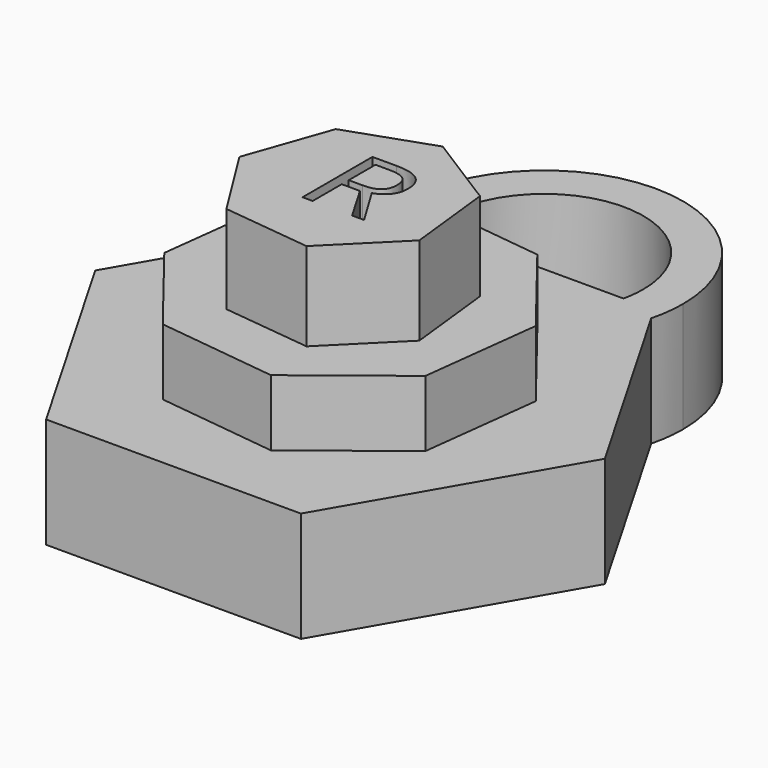
from build123d import *

# Parameters (mm, degrees)
F1_DEPTH     = 6.35
F3_DEPTH     = 3.81
F5_DEPTH     = 5.08
F6_TEXT_SIZE = 7.0421571462
F7_DEPTH     = 4.064
F9_DEPTH     = 6.35


# Not quite as in the source:
# - Text() gives the source's letters only with a copy of the font that has no kerning and outlines rounded to 1/6400 em; it was checked with that copy


with BuildPart() as f1:
    # F0 (on Top) → F1 (new body)
    with BuildSketch(Plane.XY):
        Polygon((7.3323484187, 12.7), (-7.3323484187, 12.7), (-14.6646968374, 0), (-7.3323484187, -12.7), (7.3323484187, -12.7), (14.6646968374, 0), align=None)
    extrude(amount=F1_DEPTH)

    # F2 (on face) → F3 (join)
    with BuildSketch(Plane.XY.offset(6.35)):
        Polygon((2.4380916696, -8.7388779051), (7.9033109794, -4.4553286739), (8.7388779051, 2.4380916696), (4.4553286739, 7.9033109794), (-2.4380916696, 8.7388779051), (-7.9033109794, 4.4553286739), (-8.7388779051, -2.4380916696), (-4.4553286739, -7.9033109794), align=None)
    extrude(amount=F3_DEPTH)

    # F4 (on face) → F5 (join)
    with BuildSketch(Plane.XY.offset(10.16)):
        Polygon((1.9345783961, -5.5516942813), (5.5466792711, -1.948910472), (4.9820175233, 3.1214426732), (0.6657949658, 5.8412858197), (-4.1517847807, 4.1625216035), (-5.8429859063, -0.6507062802), (-3.1342994693, -4.9739390629), align=None)
    extrude(amount=F5_DEPTH)

    # F6 (on face) → F7 (cut)
    with BuildSketch(Plane.XY.offset(15.24)):
        with Locations((-1.86573028, -1.948910472)):
            Text('R', F6_TEXT_SIZE, font='Open Sans', text_align=(TextAlign.LEFT, TextAlign.BOTTOM))
    extrude(amount=-F7_DEPTH, mode=Mode.SUBTRACT)

    # F8 (on face) → F9 (join)
    with BuildSketch(Plane(origin=(0, 0, 0), x_dir=(1, 0, 0), z_dir=(0, 0, -1))):
        with BuildLine():
            ThreePointArc((5.5739029196, -12.7), (5.6796161924, -13.3271057527), (5.715, -13.9620741829))
            ThreePointArc((5.715, -13.9620741829), (-0.6349684302, -19.6416903753), (-5.5739029196, -12.7))
            Line((-5.5739029196, -12.7), (-7.3323484187, -12.7))
            Line((-7.3323484187, -12.7), (-7.7505101922, -11.9757225625))
            ThreePointArc((-7.7505101922, -11.9757225625), (-1.0010416954, -21.9002047263), (8.001, -13.9620741829))
            ThreePointArc((8.001, -13.9620741829), (7.9381305434, -12.9610324875), (7.7505101922, -11.9757225625))
            Line((7.7505101922, -11.9757225625), (7.3323484187, -12.7))
            Line((7.3323484187, -12.7), (5.5739029196, -12.7))
        make_face()
    extrude(amount=-F9_DEPTH)


solid = f1.part
